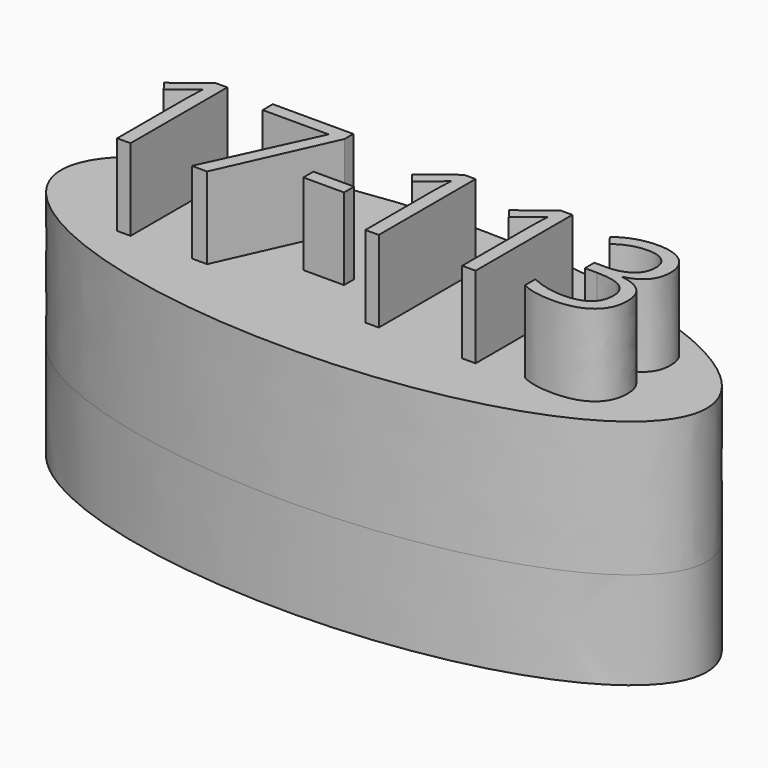
from build123d import *

# Parameters (mm, degrees)
F2_DEPTH     = 25.4
F3_DEPTH     = 35.306
F4_TEXT_SIZE = 44.3045638994
F5_DEPTH     = 21.336


# Not quite as in the source:
# - Text() gives the source's letters only with a copy of the font that has no kerning and outlines rounded to 1/6400 em; it was checked with that copy


with BuildPart() as f2:
    # F1 (on face) → F2 (new body)
    with BuildSketch(Plane.XY):
        with BuildLine():
            add(Edge.make_bspline(
                [(84.4064280391, 0), (84.4064280391, 56.7179521584), (-42.2032140195, 28.3589760792), (-168.8128560781, 0), (-42.2032140195, -28.3589760792), (84.4064280391, -56.7179521584), (84.4064280391, 0)],
                knots=[0, 0, 0, 2.0943951024, 2.0943951024, 4.1887902048, 4.1887902048, 6.2831853072, 6.2831853072, 6.2831853072], degree=2, weights=[1, 0.5, 1, 0.5, 1, 0.5, 1]))
        make_face()
    extrude(amount=F2_DEPTH)

    # F2_face (on face) + F0 (on Top) + F2_face1 (on face) → F3 (join)
    with BuildSketch(Plane(origin=(0.4482575049, 0, 25.4), x_dir=(1, 0, 0), z_dir=(0, 0, 1))):
        with BuildLine():
            add(Edge.make_bspline(
                [(83.9581705342, 0), (83.9581705342, 56.7179521584), (-42.6514715244, 28.3589760792), (-169.261113583, 0), (-42.6514715244, -28.3589760792), (83.9581705342, -56.7179521584), (83.9581705342, 0)],
                knots=[0, 0, 0, 2.0943951024, 2.0943951024, 4.1887902048, 4.1887902048, 6.2831853072, 6.2831853072, 6.2831853072], degree=2, weights=[1, 0.5, 1, 0.5, 1, 0.5, 1]))
        make_face()
    with BuildSketch(Plane.XY):
        with BuildLine():
            add(Edge.make_bspline(
                [(84.4064280391, 0), (84.4064280391, 56.7179521584), (-42.2032140195, 28.3589760792), (-168.8128560781, 0), (-42.2032140195, -28.3589760792), (84.4064280391, -56.7179521584), (84.4064280391, 0)],
                knots=[0, 0, 0, 2.0943951024, 2.0943951024, 4.1887902048, 4.1887902048, 6.2831853072, 6.2831853072, 6.2831853072], degree=2, weights=[1, 0.5, 1, 0.5, 1, 0.5, 1]))
        make_face()
    with BuildSketch(Plane(origin=(0.4482575049, 0, 0), x_dir=(1, 0, 0), z_dir=(0, 0, -1))):
        with BuildLine():
            add(Edge.make_bspline(
                [(83.9581705342, 0), (83.9581705342, -56.7179521584), (-42.6514715244, -28.3589760792), (-169.261113583, 0), (-42.6514715244, 28.3589760792), (83.9581705342, 56.7179521584), (83.9581705342, 0)],
                knots=[0, 0, 0, 2.0943951024, 2.0943951024, 4.1887902048, 4.1887902048, 6.2831853072, 6.2831853072, 6.2831853072], degree=2, weights=[1, 0.5, 1, 0.5, 1, 0.5, 1]))
        make_face()
    extrude(amount=F3_DEPTH, dir=(0, 0, 1))


with BuildPart() as f5:
    # F4 (on face) → F5 (new body)
    with BuildSketch(Plane.XY.offset(60.706)):
        with Locations((-70.5896309503, -13.9458155937)):
            Text('17-113', F4_TEXT_SIZE, font='Open Sans', text_align=(TextAlign.LEFT, TextAlign.BOTTOM))
    extrude(amount=F5_DEPTH)


solid = Compound([f2.part, f5.part])
